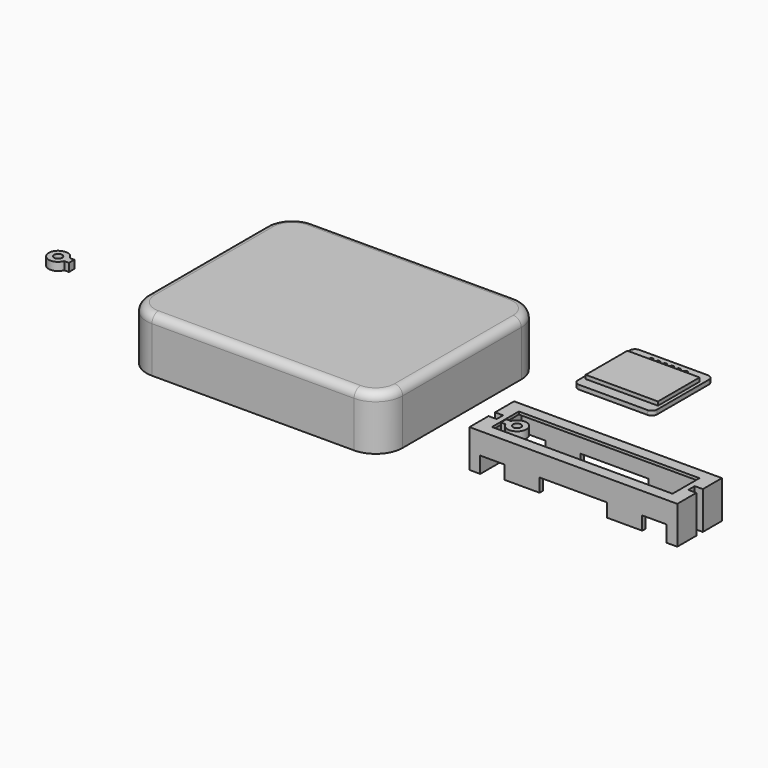
from build123d import *

# Parameters (mm, degrees)
F1_W      = 9
F1_H      = 1.6
F1_W_2    = 13
F1_W_3    = 25.1
F1_W_4    = 67
F1_H_2    = 12.5
F3_DEPTH  = 1
F4_DEPTH  = 14
F5_DEPTH  = 8
F6_DEPTH  = 13
F0_R      = 1.5
F7_DEPTH  = 3
F0_R_2    = 3.4
F8_DEPTH  = 3
F9_DEPTH  = 17
F10_R     = 3
F11_R     = 0.75
F11_W     = 26.8
F11_H     = 3.8
F12_DEPTH = 1.6
F13_DEPTH = 3
F2_R      = 3
F2_R_2    = 1
F14_DEPTH = 6


with BuildPart() as f3:
    # F1 (on face) → F3 (new body)
    with BuildSketch(Plane.XY):
        Polygon((147.9443044477, -29.0992980018), (147.9443044477, -30.6992980018), (151.9443044477, -30.6992980018), (151.9443044477, -21.8492980018), (148.9443044477, -21.8492980018), (148.9443044477, -18.8492980018), (151.9443044477, -18.8492980018), (151.9443044477, -9.9992980018), (147.9443044477, -9.9992980018), (147.9443044477, -11.5992980018), align=None)
        with Locations((83.3443044477, -29.8992980018)):
            Rectangle(F1_W, F1_H)
        with Locations((94.3443044477, -29.8992980018)):
            Rectangle(F1_W_2, F1_H)
        with Locations((113.3943044477, -29.8992980018)):
            Rectangle(F1_W_3, F1_H)
        with Locations((132.4443044477, -29.8992980018)):
            Rectangle(F1_W_2, F1_H)
        with Locations((143.4443044477, -29.8992980018)):
            Rectangle(F1_W, F1_H)
        with Locations((83.3443044477, -10.7992980018)):
            Rectangle(F1_W, F1_H)
        with Locations((94.3443044477, -10.7992980018)):
            Rectangle(F1_W_2, F1_H)
        with Locations((113.3943044477, -10.7992980018)):
            Rectangle(F1_W_3, F1_H)
        with Locations((132.4443044477, -10.7992980018)):
            Rectangle(F1_W_2, F1_H)
        with Locations((143.4443044477, -10.7992980018)):
            Rectangle(F1_W, F1_H)
        Polygon((74.8443044477, -21.8492980018), (74.8443044477, -30.6992980018), (78.8443044477, -30.6992980018), (78.8443044477, -29.0992980018), (78.8443044477, -11.5992980018), (78.8443044477, -9.9992980018), (74.8443044477, -9.9992980018), (74.8443044477, -18.8492980018), (77.8443044477, -18.8492980018), (77.8443044477, -20.3492980018), (77.8443044477, -21.8492980018), align=None)
        Polygon((78.8443044477, -11.5992980018), (78.8443044477, -29.0992980018), (87.8443044477, -29.0992980018), (100.8443044477, -29.0992980018), (125.9443044477, -29.0992980018), (138.9443044477, -29.0992980018), (147.9443044477, -29.0992980018), (147.9443044477, -11.5992980018), (138.9443044477, -11.5992980018), (125.9443044477, -11.5992980018), (100.8443044477, -11.5992980018), (87.8443044477, -11.5992980018), align=None)
        with Locations((113.3943044477, -20.3492980018)):
            Rectangle(F1_W_4, F1_H_2, mode=Mode.SUBTRACT)
    extrude(amount=-F3_DEPTH)

    # F1 (on face) → F4 (join)
    with BuildSketch(Plane.XY):
        Polygon((74.8443044477, -21.8492980018), (74.8443044477, -30.6992980018), (78.8443044477, -30.6992980018), (78.8443044477, -29.0992980018), (78.8443044477, -11.5992980018), (78.8443044477, -9.9992980018), (74.8443044477, -9.9992980018), (74.8443044477, -18.8492980018), (77.8443044477, -18.8492980018), (77.8443044477, -20.3492980018), (77.8443044477, -21.8492980018), align=None)
        Polygon((147.9443044477, -29.0992980018), (147.9443044477, -30.6992980018), (151.9443044477, -30.6992980018), (151.9443044477, -21.8492980018), (148.9443044477, -21.8492980018), (148.9443044477, -18.8492980018), (151.9443044477, -18.8492980018), (151.9443044477, -9.9992980018), (147.9443044477, -9.9992980018), (147.9443044477, -11.5992980018), align=None)
    extrude(amount=-F4_DEPTH)

    # F1 (on face) → F5 (join)
    with BuildSketch(Plane.XY):
        with Locations((83.3443044477, -29.8992980018)):
            Rectangle(F1_W, F1_H)
        with Locations((113.3943044477, -29.8992980018)):
            Rectangle(F1_W_3, F1_H)
        with Locations((143.4443044477, -29.8992980018)):
            Rectangle(F1_W, F1_H)
        with Locations((143.4443044477, -10.7992980018)):
            Rectangle(F1_W, F1_H)
        with Locations((113.3943044477, -10.7992980018)):
            Rectangle(F1_W_3, F1_H)
        with Locations((83.3443044477, -10.7992980018)):
            Rectangle(F1_W, F1_H)
    extrude(amount=-F5_DEPTH)

    # F1 (on face) → F6 (join)
    with BuildSketch(Plane.XY):
        with Locations((94.3443044477, -29.8992980018)):
            Rectangle(F1_W_2, F1_H)
        with Locations((132.4443044477, -29.8992980018)):
            Rectangle(F1_W_2, F1_H)
        with Locations((132.4443044477, -10.7992980018)):
            Rectangle(F1_W_2, F1_H)
        with Locations((94.3443044477, -10.7992980018)):
            Rectangle(F1_W_2, F1_H)
    extrude(amount=-F6_DEPTH)


with BuildPart() as f7:
    # F0 (on Top) → F7 (new body)
    with BuildSketch(Plane.XY):
        with BuildLine():
            ThreePointArc((-81.8553396934, -20.217330035), (-88.6245139011, -21.467330035), (-81.8553396934, -22.717330035))
            Line((-81.8553396934, -22.717330035), (-80.1245139011, -22.717330035))
            Line((-80.1245139011, -22.717330035), (-80.1245139011, -20.217330035))
            Line((-80.1245139011, -20.217330035), (-81.8553396934, -20.217330035))
        make_face()
        with Locations((-85.1245139011, -21.467330035)):
            Circle(F0_R, mode=Mode.SUBTRACT)
    extrude(amount=-F7_DEPTH)


with BuildPart() as f7b:
    # F0 (on Top) → F7, piece 2 (new body)
    with BuildSketch(Plane.XY):
        with BuildLine():
            Line((-47.5, 27.5), (-47.5, -27.5))
            ThreePointArc((-47.5, -27.5), (-44.5710678119, -34.5710678119), (-37.5, -37.5))
            Line((-37.5, -37.5), (37.5, -37.5))
            ThreePointArc((37.5, -37.5), (44.5710678119, -34.5710678119), (47.5, -27.5))
            Line((47.5, -27.5), (47.5, 27.5))
            ThreePointArc((47.5, 27.5), (44.5710678119, 34.5710678119), (37.5, 37.5))
            Line((37.5, 37.5), (-37.5, 37.5))
            ThreePointArc((-37.5, 37.5), (-44.5710678119, 34.5710678119), (-47.5, 27.5))
        make_face()
        with BuildLine():
            Line((37.5, -34.5), (-37.5, -34.5))
            ThreePointArc((-37.5, -34.5), (-42.4497474683, -32.4497474683), (-44.5, -27.5))
            Line((-44.5, -27.5), (-44.5, 27.5))
            ThreePointArc((-44.5, 27.5), (-42.4497474683, 32.4497474683), (-37.5, 34.5))
            Line((-37.5, 34.5), (37.5, 34.5))
            ThreePointArc((37.5, 34.5), (42.4497474683, 32.4497474683), (44.5, 27.5))
            Line((44.5, 27.5), (44.5, -27.5))
            ThreePointArc((44.5, -27.5), (42.4497474683, -32.4497474683), (37.5, -34.5))
        make_face(mode=Mode.SUBTRACT)
    extrude(amount=-F7_DEPTH)

    # F0 (on Top) → F8 (join)
    with BuildSketch(Plane.XY):
        with BuildLine():
            Line((-47.5, 27.5), (-47.5, -27.5))
            ThreePointArc((-47.5, -27.5), (-44.5710678119, -34.5710678119), (-37.5, -37.5))
            Line((-37.5, -37.5), (37.5, -37.5))
            ThreePointArc((37.5, -37.5), (44.5710678119, -34.5710678119), (47.5, -27.5))
            Line((47.5, -27.5), (47.5, 27.5))
            ThreePointArc((47.5, 27.5), (44.5710678119, 34.5710678119), (37.5, 37.5))
            Line((37.5, 37.5), (-37.5, 37.5))
            ThreePointArc((-37.5, 37.5), (-44.5710678119, 34.5710678119), (-47.5, 27.5))
        make_face()
        with BuildLine():
            Line((37.5, -34.5), (-37.5, -34.5))
            ThreePointArc((-37.5, -34.5), (-42.4497474683, -32.4497474683), (-44.5, -27.5))
            Line((-44.5, -27.5), (-44.5, 27.5))
            ThreePointArc((-44.5, 27.5), (-42.4497474683, 32.4497474683), (-37.5, 34.5))
            Line((-37.5, 34.5), (37.5, 34.5))
            ThreePointArc((37.5, 34.5), (42.4497474683, 32.4497474683), (44.5, 27.5))
            Line((44.5, 27.5), (44.5, -27.5))
            ThreePointArc((44.5, -27.5), (42.4497474683, -32.4497474683), (37.5, -34.5))
        make_face(mode=Mode.SUBTRACT)
        with BuildLine():
            ThreePointArc((-44.5, -27.5), (-42.4497474683, -32.4497474683), (-37.5, -34.5))
            Line((-37.5, -34.5), (37.5, -34.5))
            ThreePointArc((37.5, -34.5), (42.4497474683, -32.4497474683), (44.5, -27.5))
            Line((44.5, -27.5), (44.5, 27.5))
            ThreePointArc((44.5, 27.5), (42.4497474683, 32.4497474683), (37.5, 34.5))
            Line((37.5, 34.5), (-37.5, 34.5))
            ThreePointArc((-37.5, 34.5), (-42.4497474683, 32.4497474683), (-44.5, 27.5))
            Line((-44.5, 27.5), (-44.5, -27.5))
        make_face()
        with Locations((-37.1, -28.1)):
            Circle(F0_R_2, mode=Mode.SUBTRACT)
        with Locations((37.1, -28.1)):
            Circle(F0_R_2, mode=Mode.SUBTRACT)
        with Locations((-37.1, 28.1)):
            Circle(F0_R_2, mode=Mode.SUBTRACT)
        with Locations((37.1, 28.1)):
            Circle(F0_R_2, mode=Mode.SUBTRACT)
        with Locations((-37.1, -28.1)):
            Circle(F0_R_2)
        with Locations((-37.1, -28.1)):
            Circle(F0_R, mode=Mode.SUBTRACT)
        with Locations((37.1, -28.1)):
            Circle(F0_R_2)
        with Locations((37.1, -28.1)):
            Circle(F0_R, mode=Mode.SUBTRACT)
        with Locations((-37.1, 28.1)):
            Circle(F0_R_2)
        with Locations((-37.1, 28.1)):
            Circle(F0_R, mode=Mode.SUBTRACT)
        with Locations((37.1, 28.1)):
            Circle(F0_R_2)
        with Locations((37.1, 28.1)):
            Circle(F0_R, mode=Mode.SUBTRACT)
        with Locations((-37.1, -28.1)):
            Circle(F0_R)
        with Locations((37.1, -28.1)):
            Circle(F0_R)
        with Locations((-37.1, 28.1)):
            Circle(F0_R)
        with Locations((37.1, 28.1)):
            Circle(F0_R)
    extrude(amount=F8_DEPTH)

    # F0 (on Top) → F9 (join)
    with BuildSketch(Plane.XY):
        with BuildLine():
            Line((-47.5, 27.5), (-47.5, -27.5))
            ThreePointArc((-47.5, -27.5), (-44.5710678119, -34.5710678119), (-37.5, -37.5))
            Line((-37.5, -37.5), (37.5, -37.5))
            ThreePointArc((37.5, -37.5), (44.5710678119, -34.5710678119), (47.5, -27.5))
            Line((47.5, -27.5), (47.5, 27.5))
            ThreePointArc((47.5, 27.5), (44.5710678119, 34.5710678119), (37.5, 37.5))
            Line((37.5, 37.5), (-37.5, 37.5))
            ThreePointArc((-37.5, 37.5), (-44.5710678119, 34.5710678119), (-47.5, 27.5))
        make_face()
        with BuildLine():
            Line((37.5, -34.5), (-37.5, -34.5))
            ThreePointArc((-37.5, -34.5), (-42.4497474683, -32.4497474683), (-44.5, -27.5))
            Line((-44.5, -27.5), (-44.5, 27.5))
            ThreePointArc((-44.5, 27.5), (-42.4497474683, 32.4497474683), (-37.5, 34.5))
            Line((-37.5, 34.5), (37.5, 34.5))
            ThreePointArc((37.5, 34.5), (42.4497474683, 32.4497474683), (44.5, 27.5))
            Line((44.5, 27.5), (44.5, -27.5))
            ThreePointArc((44.5, -27.5), (42.4497474683, -32.4497474683), (37.5, -34.5))
        make_face(mode=Mode.SUBTRACT)
        with Locations((-37.1, -28.1)):
            Circle(F0_R_2)
        with Locations((-37.1, -28.1)):
            Circle(F0_R, mode=Mode.SUBTRACT)
        with Locations((37.1, -28.1)):
            Circle(F0_R_2)
        with Locations((37.1, -28.1)):
            Circle(F0_R, mode=Mode.SUBTRACT)
        with Locations((37.1, 28.1)):
            Circle(F0_R_2)
        with Locations((37.1, 28.1)):
            Circle(F0_R, mode=Mode.SUBTRACT)
        with Locations((-37.1, 28.1)):
            Circle(F0_R_2)
        with Locations((-37.1, 28.1)):
            Circle(F0_R, mode=Mode.SUBTRACT)
    extrude(amount=-F9_DEPTH)

    # F10
    f10_edges = [f7b.edges().sort_by_distance(p)[0] for p in [
        (-47.5, 0, 3),
        (-44.571068, -34.571068, 3),
        (0, -37.5, 3),
        (44.571068, -34.571068, 3),
        (47.5, 0, 3),
        (44.571068, 34.571068, 3),
        (0, 37.5, 3),
        (-44.571068, 34.571068, 3),
    ]]
    fillet(f10_edges, radius=F10_R)

    # F2 (on face) → F14 (join)
    with BuildSketch(Plane.XY):
        with BuildLine():
            ThreePointArc((-33, 29.7), (-35.2603520431, 32.6073907374), (-38.6352805999, 31.1336304125))
            ThreePointArc((-38.6352805999, 31.1336304125), (-35.3195441651, 30.9965457048), (-33.7, 28.1))
            ThreePointArc((-33.7, 28.1), (-33.7044453555, 27.9261936236), (-33.7177697979, 27.7528417361))
            ThreePointArc((-33.7177697979, 27.7528417361), (-33.185156256, 28.6623802735), (-33, 29.7))
        make_face()
        with Locations((26, 29.7)):
            Circle(F2_R)
        with Locations((26, 29.7)):
            Circle(F2_R_2, mode=Mode.SUBTRACT)
        with Locations((26, -7.3)):
            Circle(F2_R)
        with Locations((26, -7.3)):
            Circle(F2_R_2, mode=Mode.SUBTRACT)
        with Locations((-36, -7.3)):
            Circle(F2_R)
        with Locations((-36, -7.3)):
            Circle(F2_R_2, mode=Mode.SUBTRACT)
    extrude(amount=-F14_DEPTH)


with BuildPart() as f7c:
    # F0 (on Top) → F7, piece 3 (new body)
    with BuildSketch(Plane.XY):
        with BuildLine():
            Line((80.1245139011, -22.717330035), (81.8553396934, -22.717330035))
            ThreePointArc((81.8553396934, -22.717330035), (88.6245139011, -21.467330035), (81.8553396934, -20.217330035))
            Line((81.8553396934, -20.217330035), (80.1245139011, -20.217330035))
            Line((80.1245139011, -20.217330035), (80.1245139011, -22.717330035))
        make_face()
        with Locations((85.1245139011, -21.467330035)):
            Circle(F0_R, mode=Mode.SUBTRACT)
    extrude(amount=-F7_DEPTH)


with BuildPart() as f12:
    # F11 (on face) → F12 (new body)
    with BuildSketch(Plane.XY.offset(3)):
        with BuildLine():
            ThreePointArc((115.9400514501, 28.9685745354), (115.3542650125, 30.3827880978), (113.9400514501, 30.9685745354))
            Line((113.9400514501, 30.9685745354), (88.5400514501, 30.9685745354))
            ThreePointArc((88.5400514501, 30.9685745354), (87.1258378878, 30.3827880978), (86.5400514501, 28.9685745354))
            Line((86.5400514501, 28.9685745354), (86.5400514501, 16.6185745354))
            Line((86.5400514501, 16.6185745354), (87.8400514501, 16.6340507259))
            Line((87.8400514501, 16.6340507259), (87.8400514501, 26.2685745354))
            Line((87.8400514501, 26.2685745354), (114.6400514501, 26.2685745354))
            Line((114.6400514501, 26.2685745354), (114.6400514501, 16.9530983449))
            Line((114.6400514501, 16.9530983449), (115.9400514501, 16.9685745354))
            Line((115.9400514501, 16.9685745354), (115.9400514501, 28.9685745354))
        make_face()
        with Locations((94.8900514501, 28.4685745354)):
            Circle(F11_R, mode=Mode.SUBTRACT)
        with Locations((97.4300514501, 28.4685745354)):
            Circle(F11_R, mode=Mode.SUBTRACT)
        with Locations((99.9700514501, 28.4685745354)):
            Circle(F11_R, mode=Mode.SUBTRACT)
        with Locations((102.5100514501, 28.4685745354)):
            Circle(F11_R, mode=Mode.SUBTRACT)
        with Locations((105.0500514501, 28.4685745354)):
            Circle(F11_R, mode=Mode.SUBTRACT)
        with Locations((107.5900514501, 28.4685745354)):
            Circle(F11_R, mode=Mode.SUBTRACT)
        with BuildLine():
            Line((115.9400514501, 4.9685745354), (115.9400514501, 16.9685745354))
            Line((115.9400514501, 16.9685745354), (114.6400514501, 16.9530983449))
            Line((114.6400514501, 16.9530983449), (114.6400514501, 10.7685745354))
            Line((114.6400514501, 10.7685745354), (114.6400514501, 6.9685745354))
            Line((114.6400514501, 6.9685745354), (87.8400514501, 6.9685745354))
            Line((87.8400514501, 6.9685745354), (87.8400514501, 10.7685745354))
            Line((87.8400514501, 10.7685745354), (87.8400514501, 16.6340507259))
            Line((87.8400514501, 16.6340507259), (86.5400514501, 16.6185745354))
            Line((86.5400514501, 16.6185745354), (86.5400514501, 4.9685745354))
            ThreePointArc((86.5400514501, 4.9685745354), (87.1258378878, 3.554360973), (88.5400514501, 2.9685745354))
            Line((88.5400514501, 2.9685745354), (113.9400514501, 2.9685745354))
            ThreePointArc((113.9400514501, 2.9685745354), (115.3542650125, 3.554360973), (115.9400514501, 4.9685745354))
        make_face()
        Polygon((87.8400514501, 16.6340507259), (114.6400514501, 16.9530983449), (114.6400514501, 26.2685745354), (87.8400514501, 26.2685745354), align=None)
        Polygon((114.6400514501, 10.7685745354), (114.6400514501, 16.9530983449), (87.8400514501, 16.6340507259), (87.8400514501, 10.7685745354), align=None)
        with Locations((101.2400514501, 8.8685745354)):
            Rectangle(F11_W, F11_H)
    extrude(amount=F12_DEPTH)

    # F11 (on face) → F13 (join)
    with BuildSketch(Plane.XY.offset(3)):
        Polygon((87.8400514501, 16.6340507259), (114.6400514501, 16.9530983449), (114.6400514501, 26.2685745354), (87.8400514501, 26.2685745354), align=None)
        Polygon((114.6400514501, 10.7685745354), (114.6400514501, 16.9530983449), (87.8400514501, 16.6340507259), (87.8400514501, 10.7685745354), align=None)
        with Locations((101.2400514501, 8.8685745354)):
            Rectangle(F11_W, F11_H)
    extrude(amount=F13_DEPTH)


solid = Compound([f3.part, f7.part, f7b.part, f7c.part, f12.part])
